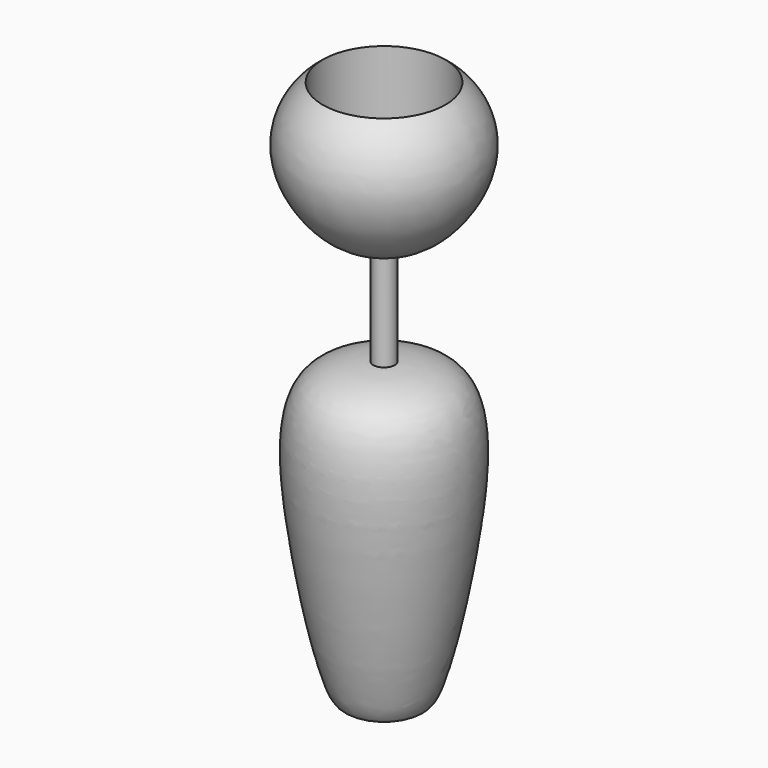
from build123d import *

# Parameters (mm, degrees)
F3_R     = 12.8249637965
F4_DEPTH = 30.4
F5_R     = 0.75
F6_DEPTH = 72


with BuildPart() as f1:
    # F0 (on Front) → F1 (revolve)
    with BuildSketch(Plane.XZ):
        with BuildLine():
            Line((0, 71.9589648982), (0, 71.956420194))
            Line((0, 71.956420194), (0, 43.3337725699))
            add(Edge.make_bspline(
                [(0, 43.3337725699), (0.6768933098, 42.5310779527), (1.4235595832, 41.9677112034), (2.2170609058, 41.6128150429)],
                knots=[0, 0, 0, 0, 0.0466672624, 0.0466672624, 0.0466672624, 0.0466672624], degree=3))
            add(Edge.make_bspline(
                [(2.2170609058, 41.6128150429), (7.914921835, 39.0644273981), (24.8773683832, 56.2108187873), (11.8622883606, 75.4374940312), (0.0647357854, 72.0839224676), (0, 71.9589648982)],
                knots=[0.0466672624, 0.0466672624, 0.0466672624, 0.0466672624, 0.3817688732, 0.747309423, 0.9958359163, 0.9958359163, 0.9958359163, 0.9958359163], degree=3))
        make_face()
        with BuildLine():
            add(Edge.make_bspline(
                [(0, 43.3337725699), (0.6768933098, 42.5310779527), (1.4235595832, 41.9677112034), (2.2170609058, 41.6128150429)],
                knots=[0, 0, 0, 0, 0.0466672624, 0.0466672624, 0.0466672624, 0.0466672624], degree=3))
            Line((0, 43.3337725699), (0, -43.0109836161))
            add(Edge.make_bspline(
                [(0, -43.0109836161), (1.9403692446, -43.4574948657), (4.6873576342, -42.6522625523), (7.8571672052, -44.4734265141), (10.8356003842, -38.8294957891), (16.3980803441, -13.1165207328), (18.7361219996, 16.8001032293), (4.7362580885, 18.8698801439), (2.3664417141, 19.0885338353), (2.2170609058, 18.8893601298)],
                knots=[0, 0, 0, 0, 0.1006535168, 0.1744949217, 0.2698143913, 0.5106129914, 0.7495537831, 0.8979870835, 0.9616249414, 0.9616249414, 0.9616249414, 0.9616249414], degree=3))
            Line((2.2170609058, 18.8893601298), (2.2170609058, 41.6128150429))
        make_face()
    revolve(axis=Axis((0, 0, 16.7866609991), (0, 0, -1)))

    # F3 (on offset) → F4 (cut)
    with BuildSketch(Plane.XY.offset(76.3)):
        Circle(F3_R)
    extrude(amount=-F4_DEPTH, mode=Mode.SUBTRACT)

    # F5 (on Top) → F6 (cut)
    with BuildSketch(Plane.XY):
        Circle(F5_R)
    extrude(amount=F6_DEPTH, mode=Mode.SUBTRACT)


solid = f1.part
